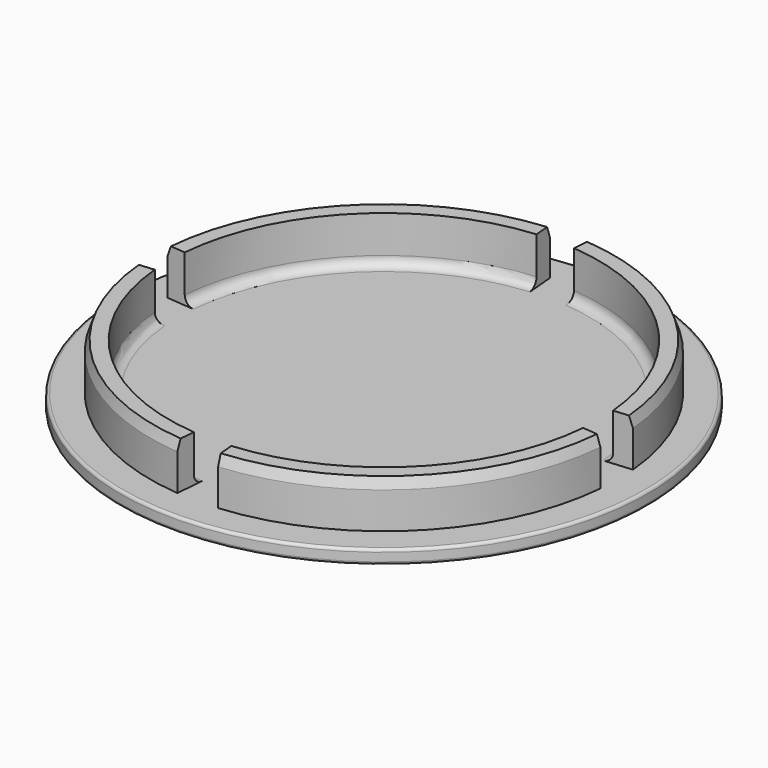
from build123d import *

# Parameters (mm, degrees)
F2_SIZE2        = 1.0989909678
F2_SIZE         = 0.4
F4_R            = 1
F3_W            = 7.3154903948
F3_H            = 6.1171914935
F5_ANGLE_BACK   = 5
F5_ANGLE        = 10
F5_COPIES_COUNT = 4
F6_R            = 0.3


# Not quite as in the source:
# - a pattern or mirror of a feature is missing from the dataset's text; its kind, count and spacing are read off the source's solid


with BuildPart() as f1:
    # F0 (on Front) → F1 (revolve)
    with BuildSketch(Plane.XZ):
        Polygon((-28.3, 0), (0, 0), (0, 1.5), (-23.05, 1.5), (-23.05, 6.5), (-25.05, 6.5), (-25.05, 1.5), (-28.3, 1.5), align=None)
    revolve(axis=Axis((0, 0, -0.5399994552), (0, 0, -1)))

    # F2
    f2_edges = [f1.edges().sort_by_distance(p)[0] for p in [
        (25.05, 0, 6.5),
    ]]
    chamfer(f2_edges, length=F2_SIZE, length2=F2_SIZE2)

    # F4
    f4_edges = [f1.edges().sort_by_distance(p)[0] for p in [
        (23.05, 0, 1.5),
    ]]
    fillet(f4_edges, radius=F4_R)

    # F3 (on Front) → F5 (revolve, cut)
    with BuildSketch(Plane.XZ, mode=Mode.PRIVATE) as f5_sk:
        with Locations((-22.2290772945, 4.5585957468)):
            Rectangle(F3_W, F3_H)
    f5 = revolve(f5_sk.sketch.rotate(Axis((0, 0, 7.0531656966), (0, 0, 1)), -F5_ANGLE_BACK), axis=Axis((0, 0, 7.0531656966), (0, 0, 1)), revolution_arc=F5_ANGLE, mode=Mode.SUBTRACT)

    # F5_copies: F5 ×4 about axis
    f5_copies_axis = Axis((0, 0, 0), (0, 0, 1))
    for i in range(1, F5_COPIES_COUNT):
        add(f5.rotate(f5_copies_axis, i * 360 / F5_COPIES_COUNT), mode=Mode.SUBTRACT)

    # F6
    f6_edges = [f1.edges().sort_by_distance(p)[0] for p in [
        (28.3, 0, 1.5),
        (28.3, 0, 0),
    ]]
    fillet(f6_edges, radius=F6_R)


solid = f1.part
